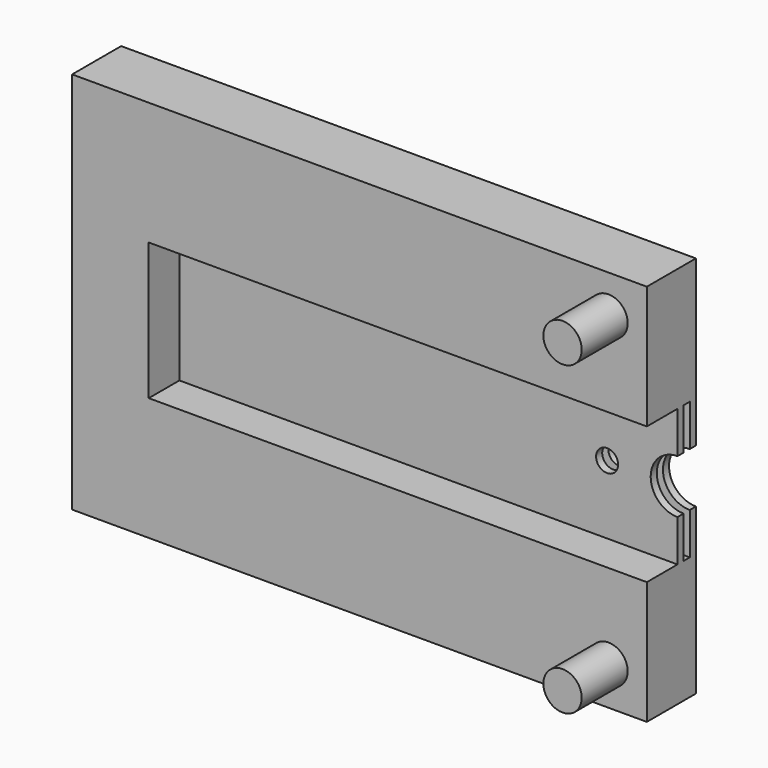
from build123d import *

# Parameters (mm, degrees)
F0_W     = 150
F0_H     = 100
F1_DEPTH = 16
F2_R     = 5
F3_DEPTH = 15
F4_W     = 130
F4_H     = 35.7704423368
F5_DEPTH = 10
F6_R     = 2.8732308489
F7_DEPTH = 7
F8_W     = 2
F8_H     = 10.8852211684
F8_H_2   = 14
F9_DEPTH = 35


with BuildPart() as f1:
    # F0 (on Front) → F1 (new body)
    with BuildSketch(Plane.XZ):
        with Locations((-201.6328409241, 45.7894764841)):
            Rectangle(F0_W, F0_H)
    extrude(amount=F1_DEPTH)

    # F2 (on face) → F3 (join)
    with BuildSketch(Plane.XZ.offset(16)):
        with Locations((-136.6328409241, 85.7894764841)):
            Circle(F2_R)
        with Locations((-136.6328409241, 5.7894764841)):
            Circle(F2_R)
    extrude(amount=F3_DEPTH)

    # F4 (on face) → F5 (cut)
    with BuildSketch(Plane.XZ.offset(16)):
        with Locations((-191.6328409241, 45.7894764841)):
            Rectangle(F4_W, F4_H)
    extrude(amount=-F5_DEPTH, mode=Mode.SUBTRACT)

    # F6 (on face) → F7 (cut)
    with BuildSketch(Plane.XZ.offset(6)):
        with Locations((-145.006071773, 45.7894764841)):
            Circle(F6_R)
        with BuildLine():
            Line((-126.6328409241, 38.7894764841), (-126.6328409241, 52.7894764841))
            ThreePointArc((-126.6328409241, 52.7894764841), (-133.6328409241, 45.7894764841), (-126.6328409241, 38.7894764841))
        make_face()
        with BuildLine():
            ThreePointArc((-126.6328409241, 38.7894764841), (-121.6830934558, 40.8397290158), (-119.6328409241, 45.7894764841))
            ThreePointArc((-119.6328409241, 45.7894764841), (-121.6830934558, 50.7392239524), (-126.6328409241, 52.7894764841))
            Line((-126.6328409241, 52.7894764841), (-126.6328409241, 38.7894764841))
        make_face()
    extrude(amount=-F7_DEPTH, mode=Mode.SUBTRACT)

    # F8 (on face) → F9 (cut)
    with BuildSketch(Plane.YZ.offset(-126.6328409241)):
        with Locations((-3, 33.3468658999)):
            Rectangle(F8_W, F8_H)
        with Locations((-3, 45.7894764841)):
            Rectangle(F8_W, F8_H_2)
        with Locations((-3, 58.2320870683)):
            Rectangle(F8_W, F8_H)
    extrude(amount=-F9_DEPTH, mode=Mode.SUBTRACT)


solid = f1.part
